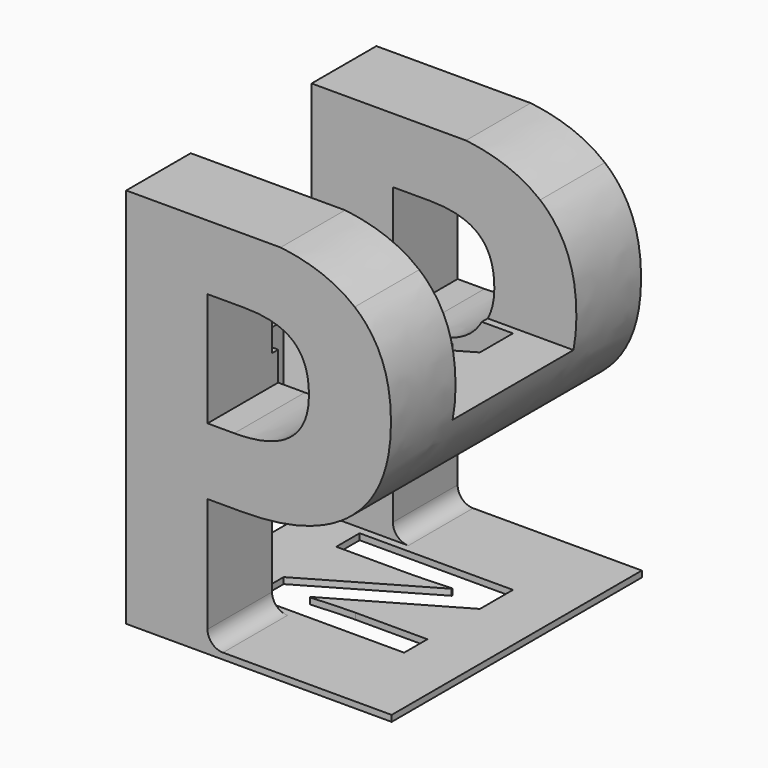
from build123d import *

# Parameters (mm, degrees)
F0_W         = 31.75
F0_H         = 31.75
F1_DEPTH     = 31.75
F3_DEPTH     = 31.751
F4_W         = 12.4067340371
F4_H         = 13.0166431847
F5_DEPTH     = 21.8005977665
F6_TEXT_SIZE = 17.6388888889
F7_DEPTH     = 31.336747925
F8_R         = 1.27


# Not quite as in the source:
# - a feature names something its author has since deleted; it is built from what else it names
# - Text() gives the source's letters only with a copy of the font that has no kerning and outlines rounded to 1/6400 em; it was checked with that copy


with BuildPart() as f1:
    # F0 (on Front) → F1 (new body)
    with BuildSketch(Plane.XZ):
        Rectangle(F0_W, F0_H)
    extrude(amount=F1_DEPTH)

    # F2 (on face) → F3 (cut, through all)
    with BuildSketch(Plane.XZ.offset(31.75)):
        with BuildLine():
            Line((-3.6449110243, -15.367), (11.4780915901, -15.367))
            Line((11.4780915901, -15.367), (11.4780915901, -15.875))
            Line((11.4780915901, -15.875), (15.875, -15.875))
            Line((15.875, -15.875), (15.875, 15.875))
            Line((15.875, 15.875), (-15.875, 15.875))
            Line((-15.875, 15.875), (-15.875, -15.875))
            Line((-15.875, -15.875), (-10.3215060764, -15.875))
            Line((-10.3215060764, -15.875), (-10.3215060764, 15.6062825521))
            Line((-10.3215060764, 15.6062825521), (-0.2687174479, 15.6062825521))
            add(Edge.make_bspline(
                [(-0.2687174479, 15.6062825521), (5.463921441, 15.6062825521), (8.4439290365, 13.139594184)],
                knots=[0, 0, 0, 1, 1, 1], degree=2))
            add(Edge.make_bspline(
                [(8.4439290365, 13.139594184), (11.4239366319, 10.672905816), (11.4239366319, 5.7877604167)],
                knots=[0, 0, 0, 1, 1, 1], degree=2))
            add(Edge.make_bspline(
                [(11.4239366319, 5.7877604167), (11.4239366319, 0.7027994792), (8.2475585938, -1.9878200955)],
                knots=[0, 0, 0, 1, 1, 1], degree=2))
            add(Edge.make_bspline(
                [(8.2475585938, -1.9878200955), (5.0711805556, -4.6784396701), (-0.7854817708, -4.6784396701)],
                knots=[0, 0, 0, 1, 1, 1], degree=2))
            Line((-0.7854817708, -4.6784396701), (-3.6449110243, -4.6784396701))
            Line((-3.6449110243, -4.6784396701), (-3.6449110243, -15.367))
        make_face()
        with BuildLine():
            Line((-3.6449110243, 10.1354709201), (-3.6449110243, 0.7923719618))
            Line((-3.6449110243, 0.7923719618), (-1.4469401042, 0.7923719618))
            add(Edge.make_bspline(
                [(-1.4469401042, 0.7923719618), (1.6260850694, 0.7923719618), (3.1557074653, 2.0084906684)],
                knots=[0, 0, 0, 1, 1, 1], degree=2))
            add(Edge.make_bspline(
                [(3.1557074653, 2.0084906684), (4.6853298611, 3.224609375), (4.6853298611, 5.5466037326)],
                knots=[0, 0, 0, 1, 1, 1], degree=2))
            add(Edge.make_bspline(
                [(4.6853298611, 5.5466037326), (4.6853298611, 7.8961588542), (3.4037543403, 9.0158148872)],
                knots=[0, 0, 0, 1, 1, 1], degree=2))
            add(Edge.make_bspline(
                [(3.4037543403, 9.0158148872), (2.1221788194, 10.1354709201), (-0.6132269965, 10.1354709201)],
                knots=[0, 0, 0, 1, 1, 1], degree=2))
            Line((-0.6132269965, 10.1354709201), (-3.6449110243, 10.1354709201))
        make_face()
    extrude(amount=-F3_DEPTH, mode=Mode.SUBTRACT)

    # F4 (on face) → F5 (cut, through all)
    with BuildSketch(Plane(origin=(-10.3215060764, 0, 0), x_dir=(0, -1, 0), z_dir=(-1, 0, 0))):
        Polygon((0, -15.875), (2.8418166706, -15.875), (2.8418166706, 15.460747825), (9.4875465114, 15.460747825), (9.4875465114, 3.1774638778), (21.8942805484, 3.1774638778), (21.8942805484, 15.460747825), (28.5194353742, 15.460747825), (28.5194353742, -15.875), (31.75, -15.875), (31.75, 15.6062825521), (0, 15.6062825521), align=None)
        with Locations((15.6909135299, -8.8586784076)):
            Rectangle(F4_W, F4_H)
    extrude(amount=-F5_DEPTH, mode=Mode.SUBTRACT)

    # F6 (on face) → F7 (cut, through all)
    with BuildSketch(Plane.XY.offset(15.460747825)):
        with Locations(Location((6.7047597991, -22.8545821711), (0, 0, 90))):
            Text('N', F6_TEXT_SIZE, font='Open Sans', font_style=FontStyle.BOLD, text_align=(TextAlign.LEFT, TextAlign.BOTTOM))
    extrude(amount=-F7_DEPTH, mode=Mode.SUBTRACT)

    # F8
    f8_edges = [f1.edges().sort_by_distance(p)[0] for p in [
        (-3.644911, -25.206858, -15.367),
        (-3.644911, -6.164682, -15.367),
    ]]
    fillet(f8_edges, radius=F8_R)


solid = f1.part
